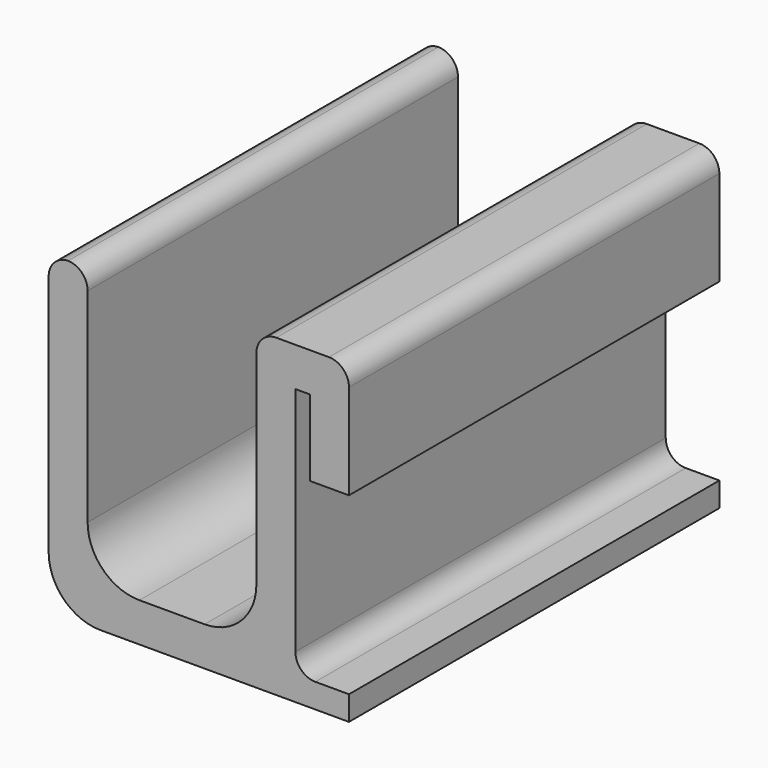
from build123d import *

# Parameters (mm, degrees)
F1_DEPTH    = 95
F2_T1_DEPTH = 95
F2_T3_DEPTH = 115.5208152802
F3_R        = 10.6225396744


# Not quite as in the source:
# - a fillet or chamfer that OpenCascade refuses, or shapes differently, is made with other operations: its cross-section is extruded or revolved along the edge and cut away or added


with BuildPart() as f1:
    # F0 (on Front) → F1 (new body)
    with BuildSketch(Plane.XZ):
        Polygon((0, 56.5581262502), (0, 0), (-34.6262017979, 0), (-34.6262017979, 56.5581262502), (-42.6262017979, 56.5581262502), (-42.6262017979, -8), (8, -8), (19, -8), (19, -3), (8, -3), (8, 48.5581262502), (11, 48.5581262502), (11, 32.9302263872), (19.0000018427, 32.9302263872), (19.0000018427, 56.5581262502), align=None)
    extrude(amount=F1_DEPTH)

    # F2: fillet of radius 4.104163056 on 5 edges, made by hand

    # F2_s2 → F2_t1 (join)
    with BuildSketch(Plane.XZ):
        with BuildLine():
            ThreePointArc((8, 1.104163056), (9.202081528, -1.797918472), (12.104163056, -3))
            Line((12.104163056, -3), (8, -3))
            Line((8, -3), (8, 1.104163056))
        make_face()
    extrude(amount=F2_T1_DEPTH)

    # F2_s4 → F2_t3 (cut)
    with BuildSketch(Plane.XZ.offset(-10.2604076401)):
        with BuildLine():
            ThreePointArc((-38.5220387419, 56.5581262502), (-41.4241202699, 55.3560447222), (-42.6262017979, 52.4539631941))
            Line((-42.6262017979, 52.4539631941), (-42.6262017979, 56.5581262502))
            Line((-42.6262017979, 56.5581262502), (-38.5220387419, 56.5581262502))
        make_face()
        with BuildLine():
            ThreePointArc((-34.6262017979, 52.4539631941), (-35.828283326, 55.3560447222), (-38.730364854, 56.5581262502))
            Line((-38.730364854, 56.5581262502), (-34.6262017979, 56.5581262502))
            Line((-34.6262017979, 56.5581262502), (-34.6262017979, 52.4539631941))
        make_face()
        with BuildLine():
            ThreePointArc((0, 52.4539631941), (1.202081528, 55.3560447222), (4.104163056, 56.5581262502))
            Line((4.104163056, 56.5581262502), (0, 56.5581262502))
            Line((0, 56.5581262502), (0, 52.4539631941))
        make_face()
        with BuildLine():
            ThreePointArc((14.8958387867, 56.5581262502), (17.7979203147, 55.3560447222), (19.0000018427, 52.4539631941))
            Line((19.0000018427, 52.4539631941), (19.0000018427, 56.5581262502))
            Line((19.0000018427, 56.5581262502), (14.8958387867, 56.5581262502))
        make_face()
    extrude(amount=F2_T3_DEPTH, mode=Mode.SUBTRACT)

    # F3
    f3_edges = [f1.edges().sort_by_distance(p)[0] for p in [
        (-34.626202, -47.5, 0),
        (0, -47.5, 0),
        (-42.626202, -47.5, -8),
    ]]
    fillet(f3_edges, radius=F3_R)


solid = f1.part
